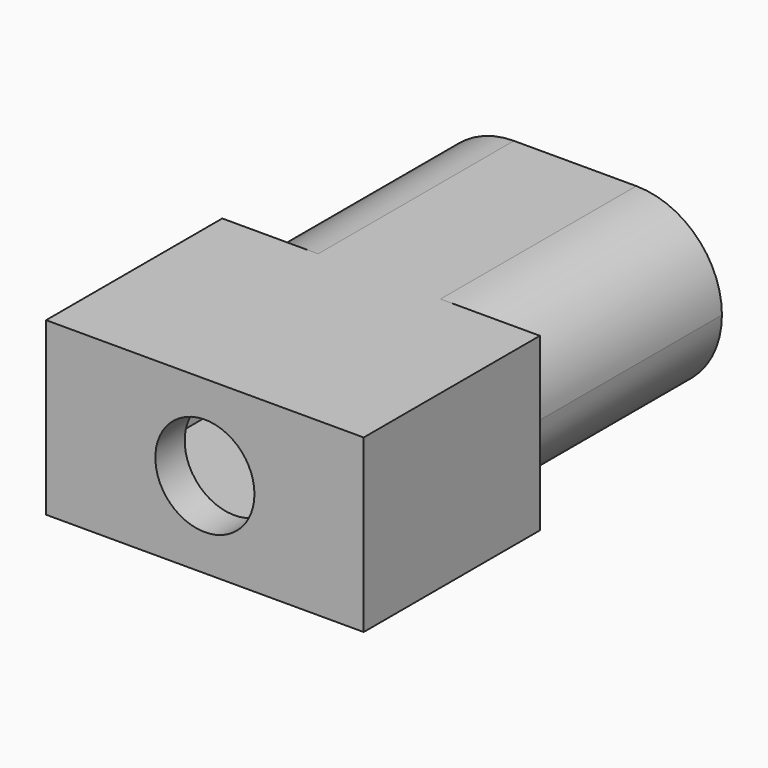
from build123d import *

# Parameters (mm, degrees)
F1_DEPTH  = 13
F2_R      = 6.8523627272
F3_DEPTH  = 30
F4_DEPTH  = 20
F5_W      = 25.9563405998
F5_H      = 14
F6_DEPTH  = 15
F7_W      = 24.6814545244
F7_H      = 12.1941640973
F8_DEPTH  = 14
F9_R      = 5.0327145122
F9_R_2    = 4.9558235457
F10_DEPTH = 3
F11_W     = 25.9563405998
F11_H     = 14
F12_DEPTH = 3
F13_R     = 4.05
F14_DEPTH = 5


with BuildPart() as f1:
    # F0 (on Front) → F1 (new body)
    with BuildSketch(Plane.XZ):
        with BuildLine():
            ThreePointArc((-21.9452433995, 6.3125732282), (-30.7452433995, 9.5621885901), (-21.9452433995, 12.8118039519))
            ThreePointArc((-21.9452433995, 12.8118039519), (-21.4056409565, 13.6804284443), (-20.7452433995, 14.4611680756))
            ThreePointArc((-20.7452433995, 14.4611680756), (-23.0334963979, 16.0155929784), (-25.7452433995, 16.5621885901))
            ThreePointArc((-25.7452433995, 16.5621885901), (-32.7452433995, 9.5621885901), (-25.7452433995, 2.5621885901))
            ThreePointArc((-25.7452433995, 2.5621885901), (-23.0334963979, 3.1087842017), (-20.7452433995, 4.6632091045))
            ThreePointArc((-20.7452433995, 4.6632091045), (-21.4056409565, 5.4439487359), (-21.9452433995, 6.3125732282))
        make_face()
        with BuildLine():
            ThreePointArc((-20.7452433995, 14.4611680756), (-20.0848458425, 13.6804284443), (-19.5452433995, 12.8118039519))
            ThreePointArc((-19.5452433995, 12.8118039519), (-14.0131925919, 14.2526043499), (-10.7452433995, 9.5621885901))
            ThreePointArc((-10.7452433995, 9.5621885901), (-14.0131925919, 4.8717728303), (-19.5452433995, 6.3125732282))
            ThreePointArc((-19.5452433995, 6.3125732282), (-20.0848458425, 5.4439487359), (-20.7452433995, 4.6632091045))
            ThreePointArc((-20.7452433995, 4.6632091045), (-18.4569904011, 3.1087842017), (-15.7452433995, 2.5621885901))
            ThreePointArc((-15.7452433995, 2.5621885901), (-10.7954959312, 4.6124411218), (-8.7452433995, 9.5621885901))
            ThreePointArc((-8.7452433995, 9.5621885901), (-10.7954959312, 14.5119360584), (-15.7452433995, 16.5621885901))
            ThreePointArc((-15.7452433995, 16.5621885901), (-18.4569904011, 16.0155929784), (-20.7452433995, 14.4611680756))
        make_face()
        with BuildLine():
            ThreePointArc((-25.7452433995, 16.5621885901), (-23.0334963979, 16.0155929784), (-20.7452433995, 14.4611680756))
            ThreePointArc((-20.7452433995, 14.4611680756), (-18.4569904011, 16.0155929784), (-15.7452433995, 16.5621885901))
            Line((-15.7452433995, 16.5621885901), (-25.7452433995, 16.5621885901))
        make_face()
        with BuildLine():
            ThreePointArc((-15.7452433995, 2.5621885901), (-18.4569904011, 3.1087842017), (-20.7452433995, 4.6632091045))
            ThreePointArc((-20.7452433995, 4.6632091045), (-23.0334963979, 3.1087842017), (-25.7452433995, 2.5621885901))
            Line((-25.7452433995, 2.5621885901), (-15.7452433995, 2.5621885901))
        make_face()
    extrude(amount=F1_DEPTH)

    # F2 (on face) → F3 (cut)
    with BuildSketch(Plane.XZ.offset(13)):
        with Locations((-20.7452433995, 9.5621885901)):
            Circle(F2_R)
    extrude(amount=-F3_DEPTH, mode=Mode.SUBTRACT)

    # F0 (on Front) → F4 (join)
    with BuildSketch(Plane.XZ):
        with BuildLine():
            ThreePointArc((-21.9452433995, 6.3125732282), (-21.0548276397, 7.8301377825), (-20.7452433995, 9.5621885901))
            ThreePointArc((-20.7452433995, 9.5621885901), (-21.0548276397, 11.2942393976), (-21.9452433995, 12.8118039519))
            ThreePointArc((-21.9452433995, 12.8118039519), (-22.7452433995, 9.5621885901), (-21.9452433995, 6.3125732282))
        make_face()
        with BuildLine():
            ThreePointArc((-19.5452433995, 6.3125732282), (-20.4356591593, 7.8301377825), (-20.7452433995, 9.5621885901))
            ThreePointArc((-20.7452433995, 9.5621885901), (-21.0548276397, 7.8301377825), (-21.9452433995, 6.3125732282))
            ThreePointArc((-21.9452433995, 6.3125732282), (-21.4056409565, 5.4439487359), (-20.7452433995, 4.6632091045))
            ThreePointArc((-20.7452433995, 4.6632091045), (-20.0848458425, 5.4439487359), (-19.5452433995, 6.3125732282))
        make_face()
        with BuildLine():
            ThreePointArc((-21.9452433995, 12.8118039519), (-21.0548276397, 11.2942393976), (-20.7452433995, 9.5621885901))
            ThreePointArc((-20.7452433995, 9.5621885901), (-20.4356591593, 11.2942393976), (-19.5452433995, 12.8118039519))
            ThreePointArc((-19.5452433995, 12.8118039519), (-20.0848458425, 13.6804284443), (-20.7452433995, 14.4611680756))
            ThreePointArc((-20.7452433995, 14.4611680756), (-21.4056409565, 13.6804284443), (-21.9452433995, 12.8118039519))
        make_face()
        with BuildLine():
            ThreePointArc((-19.5452433995, 12.8118039519), (-20.4356591593, 11.2942393976), (-20.7452433995, 9.5621885901))
            ThreePointArc((-20.7452433995, 9.5621885901), (-20.4356591593, 7.8301377825), (-19.5452433995, 6.3125732282))
            ThreePointArc((-19.5452433995, 6.3125732282), (-18.9481852123, 7.888868537), (-18.7452433995, 9.5621885901))
            ThreePointArc((-18.7452433995, 9.5621885901), (-18.9481852123, 11.2355086431), (-19.5452433995, 12.8118039519))
        make_face()
        with BuildLine():
            ThreePointArc((-21.9452433995, 6.3125732282), (-30.7452433995, 9.5621885901), (-21.9452433995, 12.8118039519))
            ThreePointArc((-21.9452433995, 12.8118039519), (-21.4056409565, 13.6804284443), (-20.7452433995, 14.4611680756))
            ThreePointArc((-20.7452433995, 14.4611680756), (-23.0334963979, 16.0155929784), (-25.7452433995, 16.5621885901))
            ThreePointArc((-25.7452433995, 16.5621885901), (-32.7452433995, 9.5621885901), (-25.7452433995, 2.5621885901))
            ThreePointArc((-25.7452433995, 2.5621885901), (-23.0334963979, 3.1087842017), (-20.7452433995, 4.6632091045))
            ThreePointArc((-20.7452433995, 4.6632091045), (-21.4056409565, 5.4439487359), (-21.9452433995, 6.3125732282))
        make_face()
        with BuildLine():
            ThreePointArc((-20.7452433995, 14.4611680756), (-20.0848458425, 13.6804284443), (-19.5452433995, 12.8118039519))
            ThreePointArc((-19.5452433995, 12.8118039519), (-14.0131925919, 14.2526043499), (-10.7452433995, 9.5621885901))
            ThreePointArc((-10.7452433995, 9.5621885901), (-14.0131925919, 4.8717728303), (-19.5452433995, 6.3125732282))
            ThreePointArc((-19.5452433995, 6.3125732282), (-20.0848458425, 5.4439487359), (-20.7452433995, 4.6632091045))
            ThreePointArc((-20.7452433995, 4.6632091045), (-18.4569904011, 3.1087842017), (-15.7452433995, 2.5621885901))
            ThreePointArc((-15.7452433995, 2.5621885901), (-10.7954959312, 4.6124411218), (-8.7452433995, 9.5621885901))
            ThreePointArc((-8.7452433995, 9.5621885901), (-10.7954959312, 14.5119360584), (-15.7452433995, 16.5621885901))
            ThreePointArc((-15.7452433995, 16.5621885901), (-18.4569904011, 16.0155929784), (-20.7452433995, 14.4611680756))
        make_face()
        with BuildLine():
            ThreePointArc((-25.7452433995, 16.5621885901), (-23.0334963979, 16.0155929784), (-20.7452433995, 14.4611680756))
            ThreePointArc((-20.7452433995, 14.4611680756), (-18.4569904011, 16.0155929784), (-15.7452433995, 16.5621885901))
            Line((-15.7452433995, 16.5621885901), (-25.7452433995, 16.5621885901))
        make_face()
        with BuildLine():
            ThreePointArc((-15.7452433995, 2.5621885901), (-18.4569904011, 3.1087842017), (-20.7452433995, 4.6632091045))
            ThreePointArc((-20.7452433995, 4.6632091045), (-23.0334963979, 3.1087842017), (-25.7452433995, 2.5621885901))
            Line((-25.7452433995, 2.5621885901), (-15.7452433995, 2.5621885901))
        make_face()
    extrude(amount=F4_DEPTH)

    # F5 (on face) → F6 (join)
    with BuildSketch(Plane.XZ.offset(20)):
        with Locations((-20.5991824623, 9.5621885901)):
            Rectangle(F5_W, F5_H)
    extrude(amount=F6_DEPTH)

    # F7 (on face) → F8 (cut)
    with BuildSketch(Plane.XZ.offset(35)):
        with Locations((-20.5570058897, 9.6122492105)):
            Rectangle(F7_W, F7_H)
    extrude(amount=-F8_DEPTH, mode=Mode.SUBTRACT)

    # F9 (on face) → F10 (cut)
    with BuildSketch(Plane.XZ.offset(21)):
        with Locations((-25.7452465594, 9.5622381195)):
            Circle(F9_R)
        with Locations((-15.7452113926, 9.5622753724)):
            Circle(F9_R_2)
    extrude(amount=-F10_DEPTH, mode=Mode.SUBTRACT)

    # F11 (on face) → F12 (join)
    with BuildSketch(Plane.XZ.offset(35)):
        with Locations((-20.5991824623, 9.5621885901)):
            Rectangle(F11_W, F11_H)
    extrude(amount=F12_DEPTH)

    # F13 (on face) → F14 (cut)
    with BuildSketch(Plane.XZ.offset(38)):
        with Locations((-20.5991824623, 9.5770442858)):
            Circle(F13_R)
    extrude(amount=-F14_DEPTH, mode=Mode.SUBTRACT)


solid = f1.part
